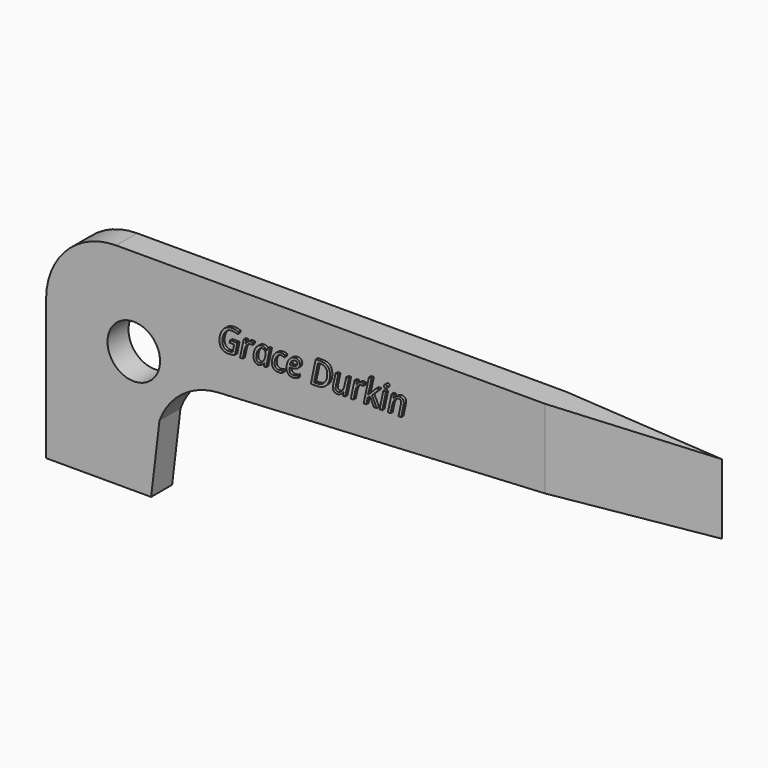
from build123d import *

# Parameters (mm, degrees)
F1_DEPTH     = 2.38125
F2_R         = 2.38125
F3_DEPTH     = 25.4
F5_DEPTH     = 25.4
F6_TEXT_SIZE = 2.9490355195
F7_DEPTH     = 0.254


# Not quite as in the source:
# - Text() gives the source's letters only with a copy of the font that has no kerning and outlines rounded to 1/6400 em; it was checked with that copy


with BuildPart() as f1:
    # F0 (on Front) → F1 (new body)
    with BuildSketch(Plane.XZ):
        with BuildLine():
            Line((60.325, 19.05), (6.35, 19.05))
            ThreePointArc((6.35, 19.05), (1.8598719395, 17.1901280605), (0, 12.7))
            Line((0, 12.7), (0, 0))
            Line((0, 0), (9.525, 0))
            Line((9.525, 0), (10.282786563, 6.3537033275))
            ThreePointArc((10.282786563, 6.3537033275), (12.3793281757, 9.1422024014), (15.6634210502, 10.3194652484))
            Line((15.6634210502, 10.3194652484), (60.325, 12.7))
            Line((60.325, 12.7), (60.325, 19.05))
        make_face()
    extrude(amount=F1_DEPTH)

    # F2 (on face) → F3 (cut)
    with BuildSketch(Plane.XZ.offset(2.38125)):
        with Locations((7.9502, 11.0998)):
            Circle(F2_R)
    extrude(amount=-F3_DEPTH, mode=Mode.SUBTRACT)

    # F4 (on face) → F5 (cut)
    with BuildSketch(Plane.XY.offset(19.05)):
        Polygon((60.325, 0), (45.24375, 0), (60.325, -1.190625), align=None)
        Polygon((60.325, -2.38125), (60.325, -1.190625), (45.24375, -2.38125), align=None)
    extrude(amount=-F5_DEPTH, mode=Mode.SUBTRACT)

    # F6 (on face) → F7 (join)
    with BuildSketch(Plane.XZ.offset(2.38125)):
        with Locations((15.7059738412, 13.9049105346)):
            Text('Grace Durkin', F6_TEXT_SIZE, font='Open Sans', font_style=FontStyle.ITALIC, text_align=(TextAlign.LEFT, TextAlign.BOTTOM))
    extrude(amount=F7_DEPTH)


solid = f1.part
